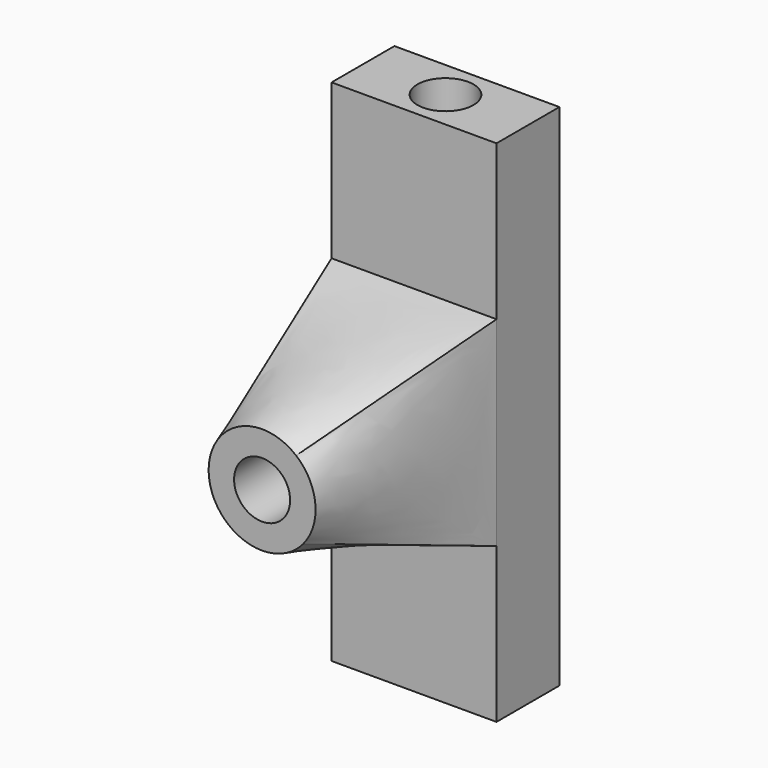
from build123d import *

# Parameters (mm, degrees)
F0_W     = 64.7669136524
F0_H     = 30.8674070984
F0_R     = 11
F1_DEPTH = 100
F4_W     = 64.7669136524
F4_H     = 78.3874105722
F6_R     = 11
F7_DEPTH = 75


# Not quite as in the source:
# - the arcs of a loft's sections are written as splines that run evenly, so that the points pair up as in the source's solid


with BuildPart() as f1:
    # F0 (on Top) → F1 (new body, symmetric)
    with BuildSketch(Plane.XY):
        Rectangle(F0_W, F0_H)
        Circle(F0_R, mode=Mode.SUBTRACT)
    extrude(amount=F1_DEPTH, both=True)

    # F4 (on face) → F5 section 0
    with BuildSketch(Plane.XZ.offset(15.4337035492)):
        Rectangle(F4_W, F4_H)
    # F3 (on offset) → F5 section 1
    with BuildSketch(Plane.XZ.offset(90)):
        with BuildLine():
            add(Edge.make_bspline(
                [(13.3759952004, 16.1889700845), (12.3164295861, 17.0644269232), (11.1706673311, 17.8355065906), (8.7506683017, 19.1393549588), (7.4764913666, 19.6720914194), (4.8486237419, 20.4787683169), (3.4949980316, 20.7526888071), (0.7602492908, 21.0311940931), (-0.6208061176, 21.0357720023), (-3.3573411141, 20.7754028748), (-4.7127530359, 20.5104622764), (-7.3459107829, 19.721224575), (-8.623591498, 19.1969469876), (-11.0521812199, 17.9091706745), (-12.203030175, 17.1457037918), (-14.3337225308, 15.4088773887), (-15.3135132459, 14.4355608147), (-16.1889700845, 13.3759952004)],
                knots=[0, 0, 0, 0, 0.125, 0.125, 0.25, 0.25, 0.375, 0.375, 0.5, 0.5, 0.625, 0.625, 0.75, 0.75, 0.875, 0.875, 1, 1, 1, 1], degree=3))
            add(Edge.make_bspline(
                [(-16.1889700845, 13.3759952004), (-17.0644269232, 12.3164295861), (-17.8355065906, 11.1706673311), (-19.1393549588, 8.7506683017), (-19.6720914194, 7.4764913666), (-20.4787683169, 4.8486237419), (-20.7526888071, 3.4949980316), (-21.0311940931, 0.7602492908), (-21.0357720023, -0.6208061176), (-20.7754028748, -3.3573411141), (-20.5104622764, -4.7127530359), (-19.721224575, -7.3459107829), (-19.1969469876, -8.623591498), (-17.9091706745, -11.0521812199), (-17.1457037918, -12.203030175), (-15.4088773887, -14.3337225308), (-14.4355608147, -15.3135132459), (-13.3759952004, -16.1889700845)],
                knots=[0, 0, 0, 0, 0.125, 0.125, 0.25, 0.25, 0.375, 0.375, 0.5, 0.5, 0.625, 0.625, 0.75, 0.75, 0.875, 0.875, 1, 1, 1, 1], degree=3))
            add(Edge.make_bspline(
                [(-13.3759952004, -16.1889700845), (-12.3164295861, -17.0644269232), (-11.1706673311, -17.8355065906), (-8.7506683017, -19.1393549588), (-7.4764913666, -19.6720914194), (-4.8486237419, -20.4787683169), (-3.4949980316, -20.7526888071), (-0.7602492908, -21.0311940931), (0.6208061176, -21.0357720023), (3.3573411141, -20.7754028748), (4.7127530359, -20.5104622764), (7.3459107829, -19.721224575), (8.623591498, -19.1969469876), (11.0521812199, -17.9091706745), (12.203030175, -17.1457037918), (14.3337225308, -15.4088773887), (15.3135132459, -14.4355608147), (16.1889700845, -13.3759952004)],
                knots=[0, 0, 0, 0, 0.125, 0.125, 0.25, 0.25, 0.375, 0.375, 0.5, 0.5, 0.625, 0.625, 0.75, 0.75, 0.875, 0.875, 1, 1, 1, 1], degree=3))
            add(Edge.make_bspline(
                [(16.1889700845, -13.3759952004), (17.0644269232, -12.3164295861), (17.8355065906, -11.1706673311), (19.1393549588, -8.7506683017), (19.6720914194, -7.4764913666), (20.4787683169, -4.8486237419), (20.7526888071, -3.4949980316), (21.0311940931, -0.7602492908), (21.0357720023, 0.6208061176), (20.7754028748, 3.3573411141), (20.5104622764, 4.7127530359), (19.721224575, 7.3459107829), (19.1969469876, 8.623591498), (17.9091706745, 11.0521812199), (17.1457037918, 12.203030175), (15.4088773887, 14.3337225308), (14.4355608147, 15.3135132459), (13.3759952004, 16.1889700845)],
                knots=[0, 0, 0, 0, 0.125, 0.125, 0.25, 0.25, 0.375, 0.375, 0.5, 0.5, 0.625, 0.625, 0.75, 0.75, 0.875, 0.875, 1, 1, 1, 1], degree=3))
        make_face()
    loft(ruled=True)

    # F6 (on face) → F7 (cut)
    with BuildSketch(Plane.XZ.offset(90)):
        Circle(F6_R)
    extrude(amount=-F7_DEPTH, mode=Mode.SUBTRACT)


solid = f1.part
